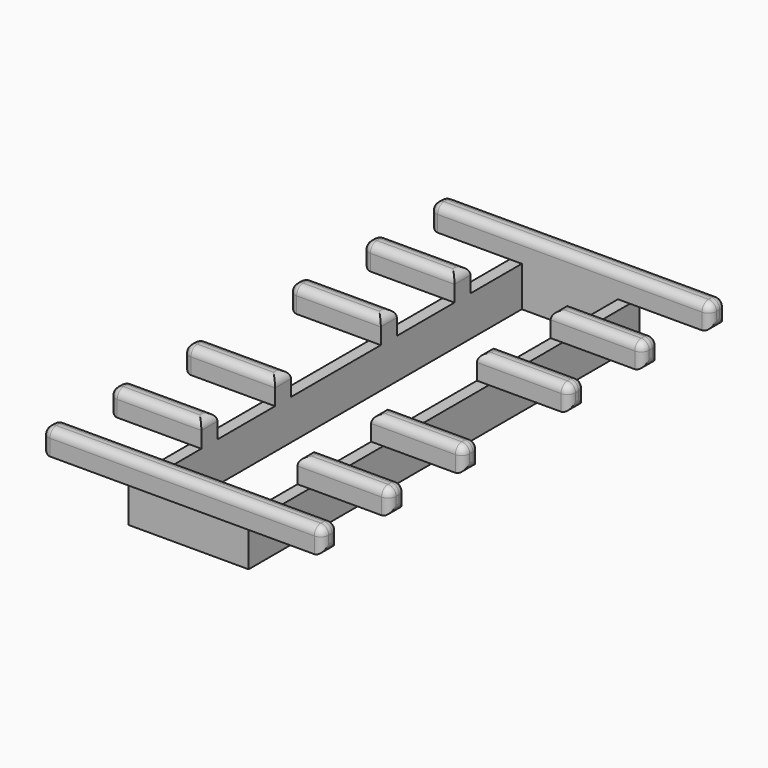
from build123d import *

# Parameters (mm, degrees)
F0_W     = 15
F0_H     = 61
F0_W_2   = 12
F0_H_2   = 58
F1_DEPTH = 5
F2_W     = 17.5
F2_H     = 2.5
F2_W_2   = 11.5
F3_DEPTH = 3
F4_R     = 1
F5_W     = 4
F5_H     = 1
F6_DEPTH = 1
F7_R     = 0.49999
F8_W     = 4
F8_H     = 1
F9_DEPTH = 1
F10_R    = 0.49999


# Not quite as in the source:
# - a fillet or chamfer is up to 0.001 mm smaller than in the source, because OpenCascade refuses the exact size


with BuildPart() as f1:
    # F0 (on Top) → F1 (new body)
    with BuildSketch(Plane.XY):
        with Locations((-39.8457739502, 26.8311633799)):
            Rectangle(F0_W, F0_H)
        with Locations((-39.8457739502, 26.8311633799)):
            Rectangle(F0_W_2, F0_H_2, mode=Mode.SUBTRACT)
    extrude(amount=F1_DEPTH)

    # F2 (on face) → F3 (join)
    with BuildSketch(Plane.XY.offset(5)):
        with Locations((-31.0957739502, 57.0811633799)):
            Rectangle(F2_W, F2_H)
        with Locations((-48.5957739502, 57.0811633799)):
            Rectangle(F2_W, F2_H)
        with Locations((-31.0957739502, -3.4188366201)):
            Rectangle(F2_W, F2_H)
        with Locations((-48.5957739502, -3.4188366201)):
            Rectangle(F2_W, F2_H)
        with Locations((-28.0957739502, 35.0811633799)):
            Rectangle(F2_W_2, F2_H)
        with Locations((-28.0957739502, 18.5811633799)):
            Rectangle(F2_W_2, F2_H)
        with Locations((-51.5957739502, 18.5811633799)):
            Rectangle(F2_W_2, F2_H)
        with Locations((-51.5957739502, 35.0811633799)):
            Rectangle(F2_W_2, F2_H)
        with Locations((-28.0957739502, 46.5811633799)):
            Rectangle(F2_W_2, F2_H)
        with Locations((-28.0957739502, 7.0811633799)):
            Rectangle(F2_W_2, F2_H)
        with Locations((-51.5957739502, 46.5811633799)):
            Rectangle(F2_W_2, F2_H)
        with Locations((-51.5957739502, 7.0811633799)):
            Rectangle(F2_W_2, F2_H)
    extrude(amount=F3_DEPTH)

    # F4
    f4_edges = [f1.edges().sort_by_distance(p)[0] for p in [
        (-22.345774, 55.831163, 6.5),
        (-22.345774, 58.331163, 6.5),
        (-22.345774, 57.081163, 5),
        (-22.345774, 57.081163, 8),
        (-22.345774, 45.331163, 6.5),
        (-22.345774, 47.831163, 6.5),
        (-22.345774, 46.581163, 5),
        (-22.345774, 46.581163, 8),
        (-22.345774, 33.831163, 6.5),
        (-22.345774, 36.331163, 6.5),
        (-22.345774, 35.081163, 5),
        (-22.345774, 35.081163, 8),
        (-22.345774, 17.331163, 6.5),
        (-22.345774, 19.831163, 6.5),
        (-22.345774, 18.581163, 5),
        (-22.345774, 18.581163, 8),
        (-22.345774, 5.831163, 6.5),
        (-22.345774, 8.331163, 6.5),
        (-22.345774, 7.081163, 5),
        (-22.345774, 7.081163, 8),
        (-22.345774, -4.668837, 6.5),
        (-22.345774, -2.168837, 6.5),
        (-22.345774, -3.418837, 5),
        (-22.345774, -3.418837, 8),
        (-45.845774, 46.581163, 8),
        (-45.845774, 35.081163, 8),
        (-45.845774, 18.581163, 8),
        (-45.845774, 7.081163, 8),
        (-57.345774, -2.168837, 6.5),
        (-57.345774, -4.668837, 6.5),
        (-57.345774, -3.418837, 5),
        (-57.345774, -3.418837, 8),
        (-57.345774, 8.331163, 6.5),
        (-57.345774, 5.831163, 6.5),
        (-57.345774, 7.081163, 5),
        (-57.345774, 7.081163, 8),
        (-57.345774, 19.831163, 6.5),
        (-57.345774, 17.331163, 6.5),
        (-57.345774, 18.581163, 5),
        (-57.345774, 18.581163, 8),
        (-57.345774, 36.331163, 6.5),
        (-57.345774, 33.831163, 6.5),
        (-57.345774, 35.081163, 5),
        (-57.345774, 35.081163, 8),
        (-57.345774, 47.831163, 6.5),
        (-57.345774, 45.331163, 6.5),
        (-57.345774, 46.581163, 5),
        (-57.345774, 46.581163, 8),
        (-57.345774, 58.331163, 6.5),
        (-57.345774, 55.831163, 6.5),
        (-57.345774, 57.081163, 5),
        (-57.345774, 57.081163, 8),
        (-33.845774, 46.581163, 8),
        (-33.845774, 35.081163, 8),
        (-33.845774, 18.581163, 8),
        (-33.845774, 7.081163, 8),
        (-39.845774, 55.831163, 8),
        (-51.595774, 45.331163, 8),
        (-28.095774, 45.331163, 8),
        (-51.595774, 33.831163, 8),
        (-28.095774, 33.831163, 8),
        (-51.595774, 17.331163, 8),
        (-28.095774, 17.331163, 8),
        (-51.595774, 5.831163, 8),
        (-28.095774, 5.831163, 8),
        (-39.845774, -4.668837, 8),
        (-39.845774, -2.168837, 8),
        (-51.595774, 8.331163, 8),
        (-28.095774, 8.331163, 8),
        (-28.095774, 19.831163, 8),
        (-51.595774, 19.831163, 8),
        (-51.595774, 36.331163, 8),
        (-28.095774, 36.331163, 8),
        (-51.595774, 47.831163, 8),
        (-28.095774, 47.831163, 8),
        (-39.845774, 58.331163, 8),
    ]]
    fillet(f4_edges, radius=F4_R)

    # F5 (on face) → F6 (join)
    with BuildSketch(Plane.YZ.offset(-32.3457739502)):
        with Locations((26.8311633799, 1)):
            Rectangle(F5_W, F5_H)
    extrude(amount=F6_DEPTH)

    # F7 (radius 0.5 in the source; OpenCascade refuses exactly that, so slightly less here)
    f7_edges = [f1.edges().sort_by_distance(p)[0] for p in [
        (-31.345774, 26.831163, 1.5),
        (-31.345774, 24.831163, 1),
        (-31.345774, 26.831163, 0.5),
        (-31.345774, 28.831163, 1),
    ]]
    fillet(f7_edges, radius=F7_R)

    # F8 (on face) → F9 (join)
    with BuildSketch(Plane(origin=(-47.3457739502, 0, 0), x_dir=(0, -1, 0), z_dir=(-1, 0, 0))):
        with Locations((-26.8311633799, 1)):
            Rectangle(F8_W, F8_H)
    extrude(amount=F9_DEPTH)

    # F10 (radius 0.5 in the source; OpenCascade refuses exactly that, so slightly less here)
    f10_edges = [f1.edges().sort_by_distance(p)[0] for p in [
        (-48.345774, 26.831163, 1.5),
        (-48.345774, 28.831163, 1),
        (-48.345774, 26.831163, 0.5),
        (-48.345774, 24.831163, 1),
    ]]
    fillet(f10_edges, radius=F10_R)


solid = f1.part
